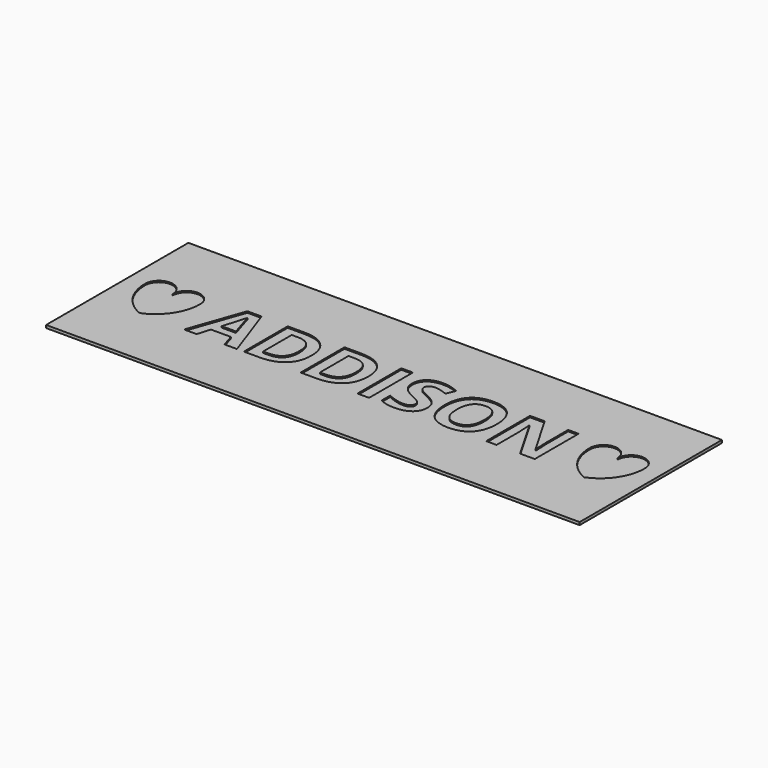
from build123d import *

# Parameters (mm, degrees)
F1_DEPTH = 0.79375
F2_W     = 3.3178445051
F2_H     = 1.541037337
F2_W_2   = 2.965173727
F3_DEPTH = 0.396875


with BuildPart() as f1:
    # F0 (on Top) → F1 (new body)
    with BuildSketch(Plane.XY):
        Polygon((76.2, 25.4), (0, 25.4), (-76.2, 25.4), (-76.2, -25.4), (76.2, -25.4), align=None)
    extrude(amount=F1_DEPTH)

    # F2 (on face) → F3 (cut)
    with BuildSketch(Plane.XY.offset(0.79375)):
        with BuildLine():
            Line((-40.3876520743, -4.1657382435), (-39.7231386171, -6.35))
            Line((-39.7231386171, -6.35), (-36.2234651266, -6.35))
            Line((-36.2234651266, -6.35), (-38.464234525, 0))
            Line((-38.464234525, 0), (-41.6121141249, 0))
            add(Edge.make_bspline(
                [(-41.1820173221, -1.385459876), (-41.4117325567, -0.6457668115), (-41.6121141249, 0)],
                knots=[0, 0, 0, 0.1461654949, 0.1461654949, 0.1461654949], degree=2))
            Line((-41.1820173221, -1.385459876), (-45.2565632056, -1.385459876))
            add(Edge.make_bspline(
                [(-44.8302608959, 0), (-45.0314281778, -0.6559669111), (-45.2565632056, -1.385459876)],
                knots=[0.8649850507, 0.8649850507, 0.8649850507, 1, 1, 1], degree=2))
            Line((-44.8302608959, 0), (-48.0257534384, 0))
            Line((-48.0257534384, 0), (-50.8, -7.891037337))
            Line((-50.8, -7.891037337), (-47.2253563846, -7.891037337))
            Line((-47.2253563846, -7.891037337), (-46.0920163111, -4.1657382435))
            Line((-46.0920163111, -4.1657382435), (-40.3876520743, -4.1657382435))
        make_face()
        Polygon((-36.2234651266, -6.35), (-39.7231386171, -6.35), (-39.2543120008, -7.891037337), (-35.6796683854, -7.891037337), align=None)
        with BuildLine():
            ThreePointArc((-63.5, -7.891037337), (-58.9819794532, -4.7535741813), (-56.2143600398, 0))
            Line((-56.2143600398, 0), (-63.5, 0))
            Line((-63.5, 0), (-63.5, -7.891037337))
        make_face()
        with BuildLine():
            Line((-63.5, 0), (-56.2143600398, 0))
            ThreePointArc((-56.2143600398, 0), (-55.7580445245, 1.9479295967), (-55.6133, 3.94335))
            ThreePointArc((-55.6133, 3.94335), (-59.55665, 7.8867), (-63.5, 3.94335))
            Line((-63.5, 3.94335), (-63.5, 0))
        make_face()
        with BuildLine():
            ThreePointArc((55.6133, 3.94335), (55.7580445245, 1.9479295967), (56.2143600398, 0))
            Line((56.2143600398, 0), (63.5, 0))
            Line((63.5, 0), (63.5, 3.94335))
            ThreePointArc((63.5, 3.94335), (59.55665, 7.8867), (55.6133, 3.94335))
        make_face()
        with BuildLine():
            Line((63.5, 0), (56.2143600398, 0))
            ThreePointArc((56.2143600398, 0), (58.9819794532, -4.7535741813), (63.5, -7.891037337))
            Line((63.5, -7.891037337), (63.5, 0))
        make_face()
        with BuildLine():
            Line((-33.7108752064, 0), (-33.7108752064, -6.35))
            Line((-33.7108752064, -6.35), (-23.5545778535, -6.35))
            add(Edge.make_bspline(
                [(-22.9304485559, -5.8366444546), (-23.2250309015, -6.1117408084), (-23.5545778535, -6.35)],
                knots=[0, 0, 0, 0.1339063994, 0.1339063994, 0.1339063994], degree=2))
            add(Edge.make_bspline(
                [(-20.7307733327, 0), (-20.7533773769, -3.8035818749), (-22.9304485559, -5.8366444546)],
                knots=[0.0103827768, 0.0103827768, 0.0103827768, 1, 1, 1], degree=2))
            Line((-20.7307733327, 0), (-24.1784936029, 0))
            add(Edge.make_bspline(
                [(-24.178492232, -0.0055926566), (-24.178492232, -0.0027955522), (-24.1784936029, 0)],
                knots=[0, 0, 0, 0.0005549689, 0.0005549689, 0.0005549689], degree=2))
            add(Edge.make_bspline(
                [(-28.9720756243, -5.1518468271), (-24.178492232, -5.1518468271), (-24.178492232, -0.0055926566)],
                knots=[0, 0, 0, 1, 1, 1], degree=2))
            Line((-28.9720756243, -5.1518468271), (-30.3930307013, -5.1518468271))
            Line((-30.3930307013, -5.1518468271), (-30.3930307013, 0))
            Line((-30.3930307013, 0), (-33.7108752064, 0))
        make_face()
        with BuildLine():
            Line((-23.5545778535, -6.35), (-33.7108752064, -6.35))
            Line((-33.7108752064, -6.35), (-33.7108752064, -7.891037337))
            Line((-33.7108752064, -7.891037337), (-29.2802345567, -7.891037337))
            add(Edge.make_bspline(
                [(-23.5545778535, -6.35), (-25.6860555689, -7.891037337), (-29.2802345567, -7.891037337)],
                knots=[0.1339063994, 0.1339063994, 0.1339063994, 1, 1, 1], degree=2))
        make_face()
        with BuildLine():
            Line((-41.6121141249, 0), (-38.464234525, 0))
            Line((-38.464234525, 0), (-41.2231051798, 7.8182202373))
            Line((-41.2231051798, 7.8182202373), (-45.2771071344, 7.8182202373))
            Line((-45.2771071344, 7.8182202373), (-48.0257534384, 0))
            Line((-48.0257534384, 0), (-44.8302608959, 0))
            add(Edge.make_bspline(
                [(-43.2364102046, 5.3871886597), (-43.5414651555, 4.2025092387), (-44.8302608959, 0)],
                knots=[0, 0, 0, 0.8649850507, 0.8649850507, 0.8649850507], degree=2))
            add(Edge.make_bspline(
                [(-42.9522191892, 4.3394482897), (-43.1508105011, 5.0037019883), (-43.2364102046, 5.3871886597)],
                knots=[0, 0, 0, 1, 1, 1], degree=2))
            add(Edge.make_bspline(
                [(-41.6121141249, 0), (-42.7826550746, 3.7722855616), (-42.9522191892, 4.3394482897)],
                knots=[0.1461654949, 0.1461654949, 0.1461654949, 1, 1, 1], degree=2))
        make_face()
        with BuildLine():
            Line((-33.7108752064, 7.7531644626), (-33.7108752064, 0))
            Line((-33.7108752064, 0), (-30.3930307013, 0))
            Line((-30.3930307013, 0), (-30.3930307013, 5.0345178816))
            Line((-30.3930307013, 5.0345178816), (-28.6296768106, 5.0345178816))
            add(Edge.make_bspline(
                [(-24.1784936029, 0), (-24.1809625009, 5.0345178816), (-28.6296768106, 5.0345178816)],
                knots=[0.0005549689, 0.0005549689, 0.0005549689, 1, 1, 1], degree=2))
            Line((-24.1784936029, 0), (-20.7307733327, 0))
            add(Edge.make_bspline(
                [(-20.7305361777, 0.0800070468), (-20.7305361777, 0.0399060776), (-20.7307733327, 0)],
                knots=[0, 0, 0, 0.0103827768, 0.0103827768, 0.0103827768], degree=2))
            add(Edge.make_bspline(
                [(-22.8499848347, 5.7312994675), (-20.7305361777, 3.7094344724), (-20.7305361777, 0.0800070468)],
                knots=[0, 0, 0, 1, 1, 1], degree=2))
            add(Edge.make_bspline(
                [(-28.8008762174, 7.7531644626), (-24.9694334917, 7.7531644626), (-22.8499848347, 5.7312994675)],
                knots=[0, 0, 0, 1, 1, 1], degree=2))
            Line((-28.8008762174, 7.7531644626), (-33.7108752064, 7.7531644626))
        make_face()
        with BuildLine():
            Line((-17.4880194116, 0), (-17.4880194116, -6.35))
            Line((-17.4880194116, -6.35), (-7.3317220587, -6.35))
            add(Edge.make_bspline(
                [(-6.7075927611, -5.8366444546), (-7.0021751067, -6.1117408084), (-7.3317220587, -6.35)],
                knots=[0, 0, 0, 0.1339063994, 0.1339063994, 0.1339063994], degree=2))
            add(Edge.make_bspline(
                [(-4.5079175379, 0), (-4.5305215821, -3.8035818749), (-6.7075927611, -5.8366444546)],
                knots=[0.0103827768, 0.0103827768, 0.0103827768, 1, 1, 1], degree=2))
            Line((-4.5079175379, 0), (-7.9556378081, 0))
            add(Edge.make_bspline(
                [(-7.9556364372, -0.0055926566), (-7.9556364372, -0.0027955522), (-7.9556378081, 0)],
                knots=[0, 0, 0, 0.0005549689, 0.0005549689, 0.0005549689], degree=2))
            add(Edge.make_bspline(
                [(-12.7492198295, -5.1518468271), (-7.9556364372, -5.1518468271), (-7.9556364372, -0.0055926566)],
                knots=[0, 0, 0, 1, 1, 1], degree=2))
            Line((-12.7492198295, -5.1518468271), (-14.1701749065, -5.1518468271))
            Line((-14.1701749065, -5.1518468271), (-14.1701749065, 0))
            Line((-14.1701749065, 0), (-17.4880194116, 0))
        make_face()
        with BuildLine():
            Line((-7.3317220587, -6.35), (-17.4880194116, -6.35))
            Line((-17.4880194116, -6.35), (-17.4880194116, -7.891037337))
            Line((-17.4880194116, -7.891037337), (-13.0573787618, -7.891037337))
            add(Edge.make_bspline(
                [(-7.3317220587, -6.35), (-9.4631997741, -7.891037337), (-13.0573787618, -7.891037337)],
                knots=[0.1339063994, 0.1339063994, 0.1339063994, 1, 1, 1], degree=2))
        make_face()
        with BuildLine():
            Line((-17.4880194116, 7.7531644626), (-17.4880194116, 0))
            Line((-17.4880194116, 0), (-14.1701749065, 0))
            Line((-14.1701749065, 0), (-14.1701749065, 5.0345178816))
            Line((-14.1701749065, 5.0345178816), (-12.4068210157, 5.0345178816))
            add(Edge.make_bspline(
                [(-7.9556378081, 0), (-7.9581067061, 5.0345178816), (-12.4068210157, 5.0345178816)],
                knots=[0.0005549689, 0.0005549689, 0.0005549689, 1, 1, 1], degree=2))
            Line((-7.9556378081, 0), (-4.5079175379, 0))
            add(Edge.make_bspline(
                [(-4.5076803828, 0.0800070468), (-4.5076803828, 0.0399060776), (-4.5079175379, 0)],
                knots=[0, 0, 0, 0.0103827768, 0.0103827768, 0.0103827768], degree=2))
            add(Edge.make_bspline(
                [(-6.6271290399, 5.7312994675), (-4.5076803828, 3.7094344724), (-4.5076803828, 0.0800070468)],
                knots=[0, 0, 0, 1, 1, 1], degree=2))
            add(Edge.make_bspline(
                [(-12.5780204226, 7.7531644626), (-8.7465776969, 7.7531644626), (-6.6271290399, 5.7312994675)],
                knots=[0, 0, 0, 1, 1, 1], degree=2))
            Line((-12.5780204226, 7.7531644626), (-17.4880194116, 7.7531644626))
        make_face()
        Polygon((-1.2651636168, 0), (-1.2651636168, -6.35), (2.0526808883, -6.35), (2.0526808883, 0), (0, 0), align=None)
        with Locations((0.3937586358, -7.1205186685)):
            Rectangle(F2_W, F2_H)
        Polygon((-1.2651636168, 7.7531644626), (-1.2651636168, 0), (0, 0), (2.0526808883, 0), (2.0526808883, 7.7531644626), align=None)
        with BuildLine():
            Line((-63.5, -7.891037337), (-63.5, 0))
            Line((-63.5, 0), (-63.5, 3.94335))
            ThreePointArc((-63.5, 3.94335), (-67.44335, 7.8867), (-71.3867, 3.94335))
            ThreePointArc((-71.3867, 3.94335), (-69.2551934305, -3.1812965916), (-63.5, -7.891037337))
        make_face()
        with BuildLine():
            Line((5.0281265797, -4.0801385401), (5.0281265797, -6.35))
            Line((5.0281265797, -6.35), (14.2588301504, -6.35))
            add(Edge.make_bspline(
                [(15.2247632528, -3.5459963907), (15.2247632528, -5.232574446), (14.2588301504, -6.35)],
                knots=[0, 0, 0, 0.7957626384, 0.7957626384, 0.7957626384], degree=2))
            add(Edge.make_bspline(
                [(14.4115660702, -0.962597341), (15.2247632528, -2.0154736933), (15.2247632528, -3.5459963907)],
                knots=[0, 0, 0, 1, 1, 1], degree=2))
            add(Edge.make_bspline(
                [(13.3789028884, 0), (14.0396930673, -0.4811196636), (14.4115660702, -0.962597341)],
                knots=[0.5427025439, 0.5427025439, 0.5427025439, 1, 1, 1], degree=2))
            Line((13.3789028884, 0), (6.9728188321, 0))
            add(Edge.make_bspline(
                [(8.9314730563, -1.1389327301), (7.6786278296, -0.5484769654), (6.9728188321, 0)],
                knots=[0, 0, 0, 0.8753644184, 0.8753644184, 0.8753644184], degree=2))
            add(Edge.make_bspline(
                [(10.9601860277, -2.1986570586), (10.4619957537, -1.8682422033), (8.9314730563, -1.1389327301)],
                knots=[0, 0, 0, 1, 1, 1], degree=2))
            add(Edge.make_bspline(
                [(11.715175412, -2.8885906683), (11.4583763017, -2.5290719139), (10.9601860277, -2.1986570586)],
                knots=[0, 0, 0, 1, 1, 1], degree=2))
            add(Edge.make_bspline(
                [(11.9719745223, -3.7069238331), (11.9719745223, -3.2481094227), (11.715175412, -2.8885906683)],
                knots=[0, 0, 0, 1, 1, 1], degree=2))
            add(Edge.make_bspline(
                [(11.3881845449, -4.9481195329), (11.9719745223, -4.5321049742), (11.9719745223, -3.7069238331)],
                knots=[0, 0, 0, 1, 1, 1], degree=2))
            add(Edge.make_bspline(
                [(9.7155663398, -5.3641340916), (10.8043945675, -5.3641340916), (11.3881845449, -4.9481195329)],
                knots=[0, 0, 0, 1, 1, 1], degree=2))
            add(Edge.make_bspline(
                [(7.7073972972, -5.0765190881), (8.8047854952, -5.3641340916), (9.7155663398, -5.3641340916)],
                knots=[0, 0, 0, 1, 1, 1], degree=2))
            add(Edge.make_bspline(
                [(5.0281265797, -4.0801385401), (6.6100090992, -4.7889040845), (7.7073972972, -5.0765190881)],
                knots=[0, 0, 0, 1, 1, 1], degree=2))
        make_face()
        with BuildLine():
            Line((14.2588301504, -6.35), (5.0281265797, -6.35))
            Line((5.0281265797, -6.35), (5.0281265797, -7.1617278637))
            add(Edge.make_bspline(
                [(9.4587672295, -8.1067485896), (6.9524079129, -8.1067485896), (5.0281265797, -7.1617278637)],
                knots=[0, 0, 0, 1, 1, 1], degree=2))
            add(Edge.make_bspline(
                [(13.6993765376, -6.8860968187), (12.1739898224, -8.1067485896), (9.4587672295, -8.1067485896)],
                knots=[0, 0, 0, 1, 1, 1], degree=2))
            add(Edge.make_bspline(
                [(14.2588301504, -6.35), (14.0109174957, -6.6367941216), (13.6993765376, -6.8860968187)],
                knots=[0.7957626384, 0.7957626384, 0.7957626384, 1, 1, 1], degree=2))
        make_face()
        with BuildLine():
            add(Edge.make_bspline(
                [(6.9728188321, 0), (6.8723247829, 0.0780928995), (6.7829205001, 0.1553347858)],
                knots=[0.8753644184, 0.8753644184, 0.8753644184, 1, 1, 1], degree=2))
            Line((6.9728188321, 0), (13.3789028884, 0))
            add(Edge.make_bspline(
                [(11.4035924915, 1.1414433694), (12.594703225, 0.5709737981), (13.3789028884, 0)],
                knots=[0, 0, 0, 0.5427025439, 0.5427025439, 0.5427025439], degree=2))
            add(Edge.make_bspline(
                [(9.3029757692, 2.2371195733), (9.746382233, 1.9323846291), (11.4035924915, 1.1414433694)],
                knots=[0, 0, 0, 1, 1, 1], degree=2))
            add(Edge.make_bspline(
                [(8.6558420113, 2.8688453847), (8.8595693054, 2.5418545176), (9.3029757692, 2.2371195733)],
                knots=[0, 0, 0, 1, 1, 1], degree=2))
            add(Edge.make_bspline(
                [(8.4521147171, 3.6341067334), (8.4521147171, 3.1958362518), (8.6558420113, 2.8688453847)],
                knots=[0, 0, 0, 1, 1, 1], degree=2))
            add(Edge.make_bspline(
                [(8.9554409733, 4.7777187713), (8.4521147171, 4.3394482897), (8.4521147171, 3.6341067334)],
                knots=[0, 0, 0, 1, 1, 1], degree=2))
            add(Edge.make_bspline(
                [(10.4003639672, 5.2159892529), (9.4587672295, 5.2159892529), (8.9554409733, 4.7777187713)],
                knots=[0, 0, 0, 1, 1, 1], degree=2))
            add(Edge.make_bspline(
                [(12.0096383918, 5.0122619587), (11.191305227, 5.2159892529), (10.4003639672, 5.2159892529)],
                knots=[0, 0, 0, 1, 1, 1], degree=2))
            add(Edge.make_bspline(
                [(14.0811512149, 4.2949364439), (12.8279715566, 4.8085346645), (12.0096383918, 5.0122619587)],
                knots=[0, 0, 0, 1, 1, 1], degree=2))
            Line((14.0811512149, 4.2949364439), (15.1494355138, 6.8766234995))
            add(Edge.make_bspline(
                [(12.8331075388, 7.688108688), (13.9407677013, 7.4004936845), (15.1494355138, 6.8766234995)],
                knots=[0, 0, 0, 1, 1, 1], degree=2))
            add(Edge.make_bspline(
                [(10.5065075995, 7.9757236916), (11.7254473764, 7.9757236916), (12.8331075388, 7.688108688)],
                knots=[0, 0, 0, 1, 1, 1], degree=2))
            add(Edge.make_bspline(
                [(6.6168570755, 6.789311802), (8.0241161999, 7.9757236916), (10.5065075995, 7.9757236916)],
                knots=[0, 0, 0, 1, 1, 1], degree=2))
            add(Edge.make_bspline(
                [(5.209597951, 3.524539113), (5.209597951, 5.6028999124), (6.6168570755, 6.789311802)],
                knots=[0, 0, 0, 1, 1, 1], degree=2))
            add(Edge.make_bspline(
                [(5.6375964682, 1.6002577798), (5.209597951, 2.4254389209), (5.209597951, 3.524539113)],
                knots=[0, 0, 0, 1, 1, 1], degree=2))
            add(Edge.make_bspline(
                [(6.7829205001, 0.1553347858), (6.0655949853, 0.7750766387), (5.6375964682, 1.6002577798)],
                knots=[0, 0, 0, 1, 1, 1], degree=2))
        make_face()
        with BuildLine():
            add(Edge.make_bspline(
                [(19.6199360487, -6.35), (19.4496608952, -6.192017507), (19.2907491659, -6.0198278199)],
                knots=[0.9174910281, 0.9174910281, 0.9174910281, 1, 1, 1], degree=2))
            Line((19.6199360487, -6.35), (30.0039240261, -6.35))
            add(Edge.make_bspline(
                [(30.3331109089, -6.0198278199), (30.1741991797, -6.192017507), (30.0039240261, -6.35)],
                knots=[0, 0, 0, 0.0825089719, 0.0825089719, 0.0825089719], degree=2))
            add(Edge.make_bspline(
                [(32.2591042362, -0.0466805143), (32.2591042362, -3.9329070502), (30.3331109089, -6.0198278199)],
                knots=[0, 0, 0, 1, 1, 1], degree=2))
            add(Edge.make_bspline(
                [(32.2590353694, 0), (32.2591042362, -0.0233075207), (32.2591042362, -0.0466805143)],
                knots=[0.9939962635, 0.9939962635, 0.9939962635, 1, 1, 1], degree=2))
            Line((32.2590353694, 0), (28.7802548956, 0))
            add(Edge.make_bspline(
                [(28.7803322886, -0.0466805143), (28.7803322886, -0.0232884716), (28.7802548956, 0)],
                knots=[0, 0, 0, 0.0044276162, 0.0044276162, 0.0044276162], degree=2))
            add(Edge.make_bspline(
                [(24.8119300374, -5.323046234), (28.7803322886, -5.323046234), (28.7803322886, -0.0466805143)],
                knots=[0, 0, 0, 1, 1, 1], degree=2))
            add(Edge.make_bspline(
                [(21.8381963401, -3.9962508307), (22.832864894, -5.323046234), (24.8119300374, -5.323046234)],
                knots=[0, 0, 0, 1, 1, 1], degree=2))
            add(Edge.make_bspline(
                [(20.8435277862, -0.0466805143), (20.8435277862, -2.6694554275), (21.8381963401, -3.9962508307)],
                knots=[0, 0, 0, 1, 1, 1], degree=2))
            add(Edge.make_bspline(
                [(20.8436079305, 0), (20.8435277862, -0.0232889211), (20.8435277862, -0.0466805143)],
                knots=[0.9910696986, 0.9910696986, 0.9910696986, 1, 1, 1], degree=2))
            Line((20.8436079305, 0), (17.3647774808, 0))
            add(Edge.make_bspline(
                [(17.3647558386, -0.0261365854), (17.3647558386, -0.0130579417), (17.3647774808, 0)],
                knots=[0, 0, 0, 0.0033476868, 0.0033476868, 0.0033476868], degree=2))
            add(Edge.make_bspline(
                [(19.2907491659, -6.0198278199), (17.3647558386, -3.9329070502), (17.3647558386, -0.0261365854)],
                knots=[0, 0, 0, 1, 1, 1], degree=2))
        make_face()
        with BuildLine():
            Line((30.0039240261, -6.35), (19.6199360487, -6.35))
            add(Edge.make_bspline(
                [(24.8119300374, -8.1067485896), (21.5133777211, -8.1067485896), (19.6199360487, -6.35)],
                knots=[0, 0, 0, 0.9174910281, 0.9174910281, 0.9174910281], degree=2))
            add(Edge.make_bspline(
                [(30.0039240261, -6.35), (28.1104823537, -8.1067485896), (24.8119300374, -8.1067485896)],
                knots=[0.0825089719, 0.0825089719, 0.0825089719, 1, 1, 1], degree=2))
        make_face()
        with BuildLine():
            add(Edge.make_bspline(
                [(17.3647774808, 0), (17.3712206547, 3.8875285368), (19.2958851481, 5.9401627439)],
                knots=[0.0033476868, 0.0033476868, 0.0033476868, 1, 1, 1], degree=2))
            Line((17.3647774808, 0), (20.8436079305, 0))
            add(Edge.make_bspline(
                [(21.8484683045, 3.9046017962), (20.8525022079, 2.5845649595), (20.8436079305, 0)],
                knots=[0, 0, 0, 0.9910696986, 0.9910696986, 0.9910696986], degree=2))
            add(Edge.make_bspline(
                [(24.8324739662, 5.2365331817), (22.8534088228, 5.2365331817), (21.8484683045, 3.9046017962)],
                knots=[0, 0, 0, 1, 1, 1], degree=2))
            add(Edge.make_bspline(
                [(28.7802548956, 0), (28.7628526871, 5.2365331817), (24.8324739662, 5.2365331817)],
                knots=[0.0044276162, 0.0044276162, 0.0044276162, 1, 1, 1], degree=2))
            Line((28.7802548956, 0), (32.2590353694, 0))
            add(Edge.make_bspline(
                [(30.3485188555, 5.9230428032), (32.247633585, 3.8588616501), (32.2590353694, 0)],
                knots=[0, 0, 0, 0.9939962635, 0.9939962635, 0.9939962635], degree=2))
            add(Edge.make_bspline(
                [(24.8324739662, 7.9996916085), (28.4379334749, 7.9996916085), (30.3485188555, 5.9230428032)],
                knots=[0, 0, 0, 1, 1, 1], degree=2))
            add(Edge.make_bspline(
                [(19.2958851481, 5.9401627439), (21.2270144576, 7.9996916085), (24.8324739662, 7.9996916085)],
                knots=[0, 0, 0, 1, 1, 1], degree=2))
        make_face()
        with BuildLine():
            Line((35.5016210023, 0), (35.5016210023, -6.35))
            Line((35.5016210023, -6.35), (38.4667947292, -6.35))
            Line((38.4667947292, -6.35), (38.4667947292, -0.5294628416))
            add(Edge.make_bspline(
                [(38.4603733247, 0), (38.4667947292, -0.2927715539), (38.4667947292, -0.5294628416)],
                knots=[0.8232036626, 0.8232036626, 0.8232036626, 1, 1, 1], degree=2))
            Line((38.4603733247, 0), (35.5016210023, 0))
        make_face()
        with Locations((36.9842078657, -7.1205186685)):
            Rectangle(F2_W_2, F2_H)
        with BuildLine():
            Line((35.5016210023, 7.7531644626), (35.5016210023, 0))
            Line((35.5016210023, 0), (38.4603733247, 0))
            add(Edge.make_bspline(
                [(38.261355441, 3.9422656658), (38.4304738155, 1.3632104543), (38.4603733247, 0)],
                knots=[0, 0, 0, 0.8232036626, 0.8232036626, 0.8232036626], degree=2))
            Line((38.261355441, 3.9422656658), (38.3572271088, 3.9422656658))
            Line((38.3572271088, 3.9422656658), (40.6249424281, 0))
            Line((40.6249424281, 0), (44.180847976, 0))
            Line((44.180847976, 0), (39.6857345061, 7.7531644626))
            Line((39.6857345061, 7.7531644626), (35.5016210023, 7.7531644626))
        make_face()
        with BuildLine():
            Line((40.6249424281, 0), (44.2776623355, -6.35))
            Line((44.2776623355, -6.35), (45.1641155259, -7.891037337))
            Line((45.1641155259, -7.891037337), (49.379044923, -7.891037337))
            Line((49.379044923, -7.891037337), (49.379044923, 0))
            Line((49.379044923, 0), (46.3958974743, 0))
            add(Edge.make_bspline(
                [(46.5542547097, -3.9637229434), (46.4136648398, -1.2984979627), (46.3958974743, 0)],
                knots=[0, 0, 0, 0.8736227194, 0.8736227194, 0.8736227194], degree=2))
            Line((46.5542547097, -3.9637229434), (46.4789269706, -3.9637229434))
            Line((46.4789269706, -3.9637229434), (44.180847976, 0))
            Line((44.180847976, 0), (40.6249424281, 0))
        make_face()
        with BuildLine():
            Line((46.3958974743, 0), (49.379044923, 0))
            Line((49.379044923, 0), (49.379044923, 7.7531644626))
            Line((49.379044923, 7.7531644626), (46.3933272672, 7.7531644626))
            Line((46.3933272672, 7.7531644626), (46.3933272672, 0.3470781215))
            add(Edge.make_bspline(
                [(46.3958974743, 0), (46.3933272672, 0.1878392556), (46.3933272672, 0.3470781215)],
                knots=[0.8736227194, 0.8736227194, 0.8736227194, 1, 1, 1], degree=2))
        make_face()
        with BuildLine():
            Line((63.5, 3.94335), (63.5, 0))
            Line((63.5, 0), (63.5, -7.891037337))
            ThreePointArc((63.5, -7.891037337), (69.2551934305, -3.1812965916), (71.3867, 3.94335))
            ThreePointArc((71.3867, 3.94335), (67.44335, 7.8867), (63.5, 3.94335))
        make_face()
    extrude(amount=-F3_DEPTH, mode=Mode.SUBTRACT)


solid = f1.part
